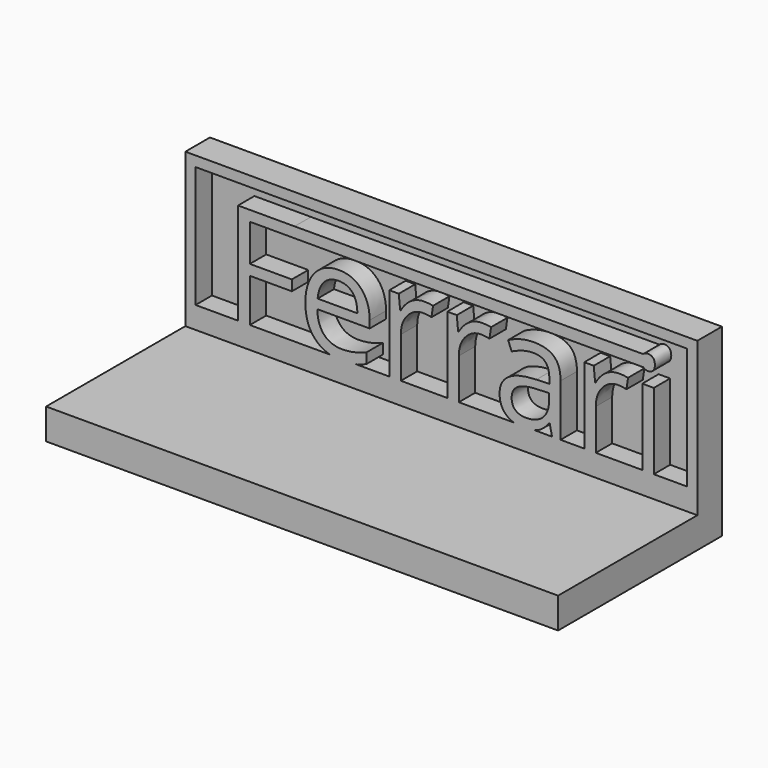
from build123d import *

# Parameters (mm, degrees)
F0_W         = 127
F0_H         = 50.8
F1_DEPTH     = 7.62
F2_T         = -2.54
F3_W         = 127
F3_H         = 7.62
F4_DEPTH     = 38.1
F5_T         = -2.54
F6_TEXT_SIZE = 35.2304571101
F7_DEPTH     = 5.08
F9_DEPTH     = 5.08
F11_DEPTH    = 5.08


# Not quite as in the source:
# - a shell that OpenCascade refuses in one call is made with other operations: the cavity is built on its own and cut out
# - Text() gives the source's letters only with a copy of the font that has no kerning and outlines rounded to 1/6400 em; it was checked with that copy


with BuildPart() as f1:
    # F0 (on Top) → F1 (new body)
    with BuildSketch(Plane.XY):
        Rectangle(F0_W, F0_H)
    extrude(amount=F1_DEPTH)

    # F2
    f2_openings = [f1.faces().sort_by_distance(p)[0] for p in [
        (0, 0, 0),
    ]]
    offset(amount=F2_T, openings=f2_openings)

    # F3 (on face) → F4 (join)
    with BuildSketch(Plane.XY.offset(7.62)):
        with Locations((0, 21.59)):
            Rectangle(F3_W, F3_H)
    extrude(amount=F4_DEPTH)

    # F5: a shell. OpenCascade refuses it in one call, so the cavity is built on its own and cut out:
    # the body offset inwards by the wall thickness, plus a prism from it out through each open face.
    f5_core = offset(f1.part, amount=F5_T, kind=Kind.INTERSECTION, mode=Mode.PRIVATE)
    f5_exits = [f5_core.faces().sort_by_distance(p)[0] for p in [
        (0, 20.32, 25.4),
    ]]
    add(f5_core, mode=Mode.SUBTRACT)
    extrude(f5_exits, amount=-F5_T, mode=Mode.SUBTRACT)

    # F6 (on face) → F7 (join)
    with BuildSketch(Plane.XZ.offset(-22.86)):
        with Locations((-53.8858510554, 13.0634428933)):
            Text('Ferrari', F6_TEXT_SIZE, font='Open Sans', text_align=(TextAlign.LEFT, TextAlign.BOTTOM))
    extrude(amount=F7_DEPTH)

    # F8 (on face) → F9 (join)
    with BuildSketch(Plane.XZ.offset(-22.86)):
        Polygon((60.96, 13.0634428933), (-50.4288624515, 13.0634428933), (-60.96, 13.0634428933), (-60.96, 7.62), (60.96, 7.62), align=None)
    extrude(amount=F9_DEPTH)

    # F10 (on face) → F11 (join)
    with BuildSketch(Plane.XZ.offset(-22.86)):
        with BuildLine():
            Line((50.0589882877, 38.4476506768), (-36.4082414734, 38.2146864146))
            Line((-36.4082414734, 38.2146864146), (-36.4082414734, 35.6164402027))
            Line((-36.4082414734, 35.6164402027), (50.0735194633, 35.5896582013))
            add(Edge.make_bspline(
                [(49.5926071878, 37.0256584871), (49.5926071878, 36.0630801012), (50.0735194633, 35.5896582013)],
                knots=[0, 0, 0, 0.9992168587, 0.9992168587, 0.9992168587], degree=2))
            add(Edge.make_bspline(
                [(50.0589882877, 38.4476506768), (49.5926071878, 37.9898328933), (49.5926071878, 37.0256584871)],
                knots=[6.8038738164, 6.8038738164, 6.8038738164, 7.7878787879, 7.7878787879, 7.7878787879], degree=2))
        make_face()
    extrude(amount=F11_DEPTH)


solid = f1.part
